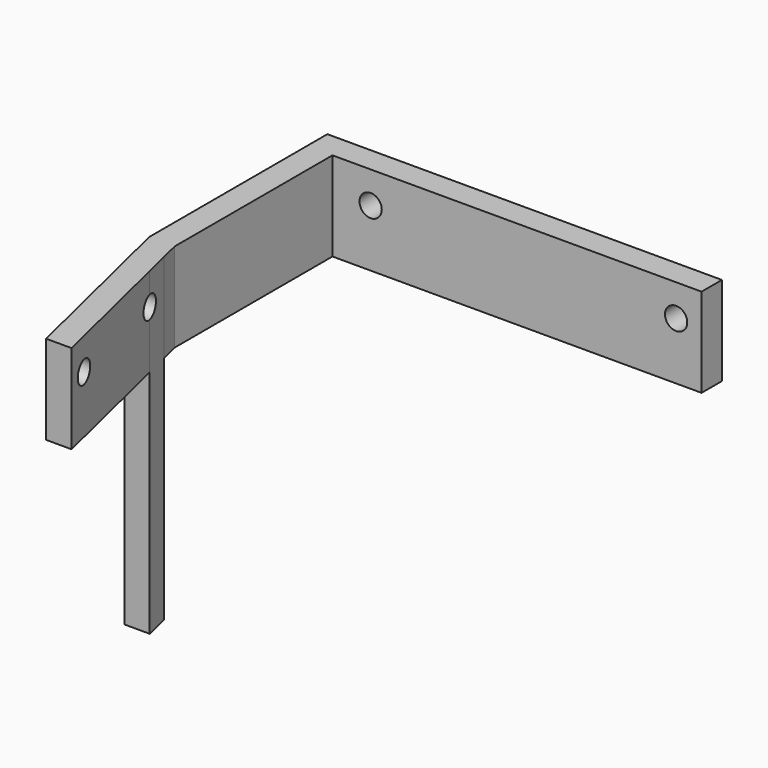
from build123d import *

# Parameters (mm, degrees)
F0_R     = 1.75
F1_DEPTH = 4
F4_DEPTH = 14
F6_DEPTH = 50.2
F5_R     = 1.75
F7_DEPTH = 71


# Not quite as in the source:
# - a feature names something its author has since deleted; it is built from what else it names


with BuildPart() as f1:
    # F0 (on Front) → F1 (new body)
    with BuildSketch(Plane.XZ):
        Polygon((-6, 5), (-6, 0), (-6, -9), (52, -9), (52, 0), (52, 5), align=None)
        Circle(F0_R, mode=Mode.SUBTRACT)
        with Locations((48, 0)):
            Circle(F0_R, mode=Mode.SUBTRACT)
    extrude(amount=F1_DEPTH)

    # F3 (on face) → F4 (join)
    with BuildSketch(Plane.XY.offset(5)):
        Polygon((-10, 0), (-10, -35), (-6, -35), (-6, -4), (-6, 0), align=None)
        Polygon((-6, -35), (-10, -35), (-9.275862069, -38), (-6, -38), align=None)
        Polygon((-5.275862069, -38), (-6, -35), (-6, -38), align=None)
        Polygon((-6, -38), (-9.275862069, -38), (-8.3103448276, -42), (-6, -42), align=None)
        Polygon((-4.3103448276, -42), (-5.275862069, -38), (-6, -38), (-6, -42), align=None)
        Polygon((-6, -42), (-8.3103448276, -42), (-6, -51.5714285714), align=None)
        Polygon((1, -64), (-4.3103448276, -42), (-6, -42), (-6, -51.5714285714), (-3, -64), align=None)
    extrude(amount=-F4_DEPTH)

    # F3 (on face) → F6 (join)
    with BuildSketch(Plane.XY.offset(5)):
        Polygon((-6, -38), (-9.275862069, -38), (-8.3103448276, -42), (-6, -42), align=None)
        Polygon((-4.3103448276, -42), (-5.275862069, -38), (-6, -38), (-6, -42), align=None)
    extrude(amount=-F6_DEPTH)

    # F5 (on face) → F7 (cut)
    with BuildSketch(Plane(origin=(-10, 0, 0), x_dir=(0, -1, 0), z_dir=(-1, 0, 0))):
        with Locations((42, 0)):
            Circle(F5_R)
        with Locations((60.5, 0)):
            Circle(F5_R)
    extrude(amount=-F7_DEPTH, mode=Mode.SUBTRACT)


solid = f1.part
